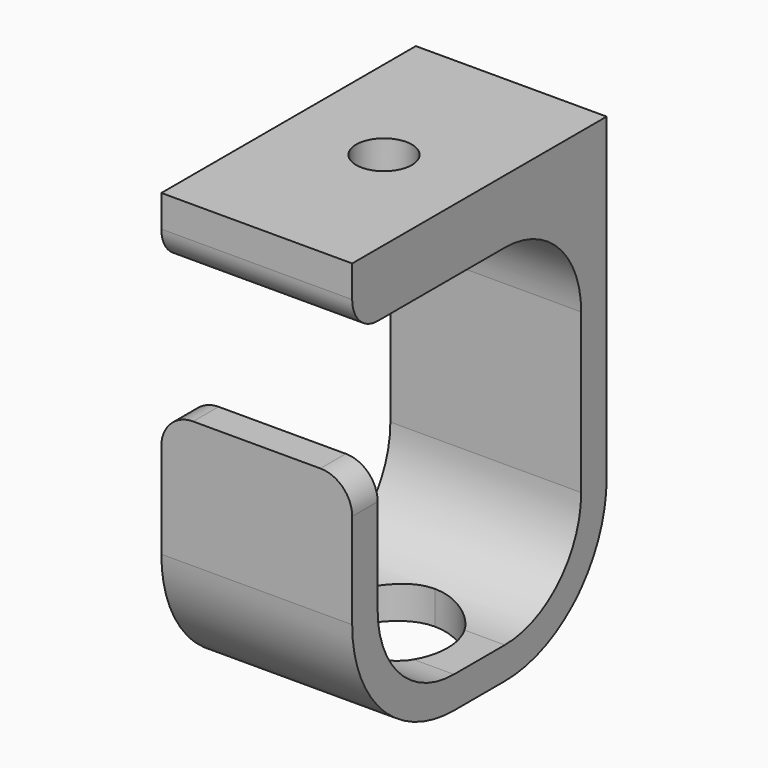
from build123d import *

# Parameters (mm, degrees)
F0_W     = 3.175
F0_H     = 6.35
F1_DEPTH = 9.525
F2_W     = 12.7
F2_H     = 6.35
F2_H_2   = 3.175
F3_DEPTH = 3.7207438789
F4_R     = 6.34999
F5_R     = 3.175
F6_R     = 2.778125
F7_DEPTH = 6.35
F8_R     = 2.778125
F9_DEPTH = 1.5875


# Not quite as in the source:
# - a fillet or chamfer is up to 0.001 mm smaller than in the source, because OpenCascade refuses the exact size
# - a feature names something its author has since deleted; it is built from what else it names


with BuildPart() as f1:
    # F0 (on Right) → F1 (new body, symmetric)
    with BuildSketch(Plane.YZ):
        with BuildLine():
            Line((31.75, 44.45), (3.175, 44.45))
            Line((3.175, 44.45), (3.175, 38.1))
            Line((3.175, 38.1), (19.05, 38.1))
            Line((19.05, 38.1), (28.575, 38.1))
            Line((28.575, 38.1), (28.575, 28.575))
            Line((28.575, 28.575), (28.575, 12.7))
            Line((28.575, 12.7), (28.575, 4.2997395874))
            ThreePointArc((28.575, 4.2997395874), (30.929762203, 8.2098719395), (31.75, 12.7))
            Line((31.75, 12.7), (31.75, 44.45))
        make_face()
        with Locations((1.5875, 41.275)):
            Rectangle(F0_W, F0_H)
        with BuildLine():
            Line((28.575, 38.1), (19.05, 38.1))
            ThreePointArc((19.05, 38.1), (25.7851920908, 35.3101920908), (28.575, 28.575))
            Line((28.575, 28.575), (28.575, 38.1))
        make_face()
        with BuildLine():
            ThreePointArc((27.4502604126, 3.175), (28.0302561211, 3.7197438789), (28.575, 4.2997395874))
            Line((28.575, 4.2997395874), (28.575, 12.7))
            ThreePointArc((28.575, 12.7), (25.7851920908, 5.9648079092), (19.05, 3.175))
            Line((19.05, 3.175), (27.4502604126, 3.175))
        make_face()
        with BuildLine():
            ThreePointArc((19.05, 0), (23.5401280605, 0.820237797), (27.4502604126, 3.175))
            Line((27.4502604126, 3.175), (19.05, 3.175))
            Line((19.05, 3.175), (12.7, 3.175))
            Line((12.7, 3.175), (4.2997395874, 3.175))
            ThreePointArc((4.2997395874, 3.175), (8.2098719395, 0.820237797), (12.7, 0))
            Line((12.7, 0), (19.05, 0))
        make_face()
        with BuildLine():
            ThreePointArc((12.7, 3.175), (5.9648079092, 5.9648079092), (3.175, 12.7))
            Line((3.175, 12.7), (3.175, 4.2997395874))
            ThreePointArc((3.175, 4.2997395874), (3.7197438789, 3.7197438789), (4.2997395874, 3.175))
            Line((4.2997395874, 3.175), (12.7, 3.175))
        make_face()
        with BuildLine():
            Line((3.175, 25.4), (0, 25.4))
            Line((0, 25.4), (0, 12.7))
            ThreePointArc((0, 12.7), (0.820237797, 8.2098719395), (3.175, 4.2997395874))
            Line((3.175, 4.2997395874), (3.175, 12.7))
            Line((3.175, 12.7), (3.175, 25.4))
        make_face()
    extrude(amount=F1_DEPTH, both=True)

    # F2 (on face) → F3 (cut, through all)
    with BuildSketch(Plane(origin=(0, 0, 0), x_dir=(1, 0, 0), z_dir=(0, 0, -1))):
        with Locations((0, -15.875)):
            Rectangle(F2_W, F2_H)
        with Locations((0, -11.1125)):
            Rectangle(F2_W, F2_H_2)
        with Locations((0, -20.6375)):
            Rectangle(F2_W, F2_H_2)
    extrude(amount=-F3_DEPTH, mode=Mode.SUBTRACT)

    # F4 (radius 6.35 in the source; OpenCascade refuses exactly that, so slightly less here)
    f4_edges = [f1.edges().sort_by_distance(p)[0] for p in [
        (-6.35, 22.225, 2.061511),
        (-6.35, 9.525, 2.061511),
        (6.35, 9.525, 2.061511),
        (6.35, 22.225, 2.061511),
    ]]
    fillet(f4_edges, radius=F4_R)

    # F5
    f5_edges = [f1.edges().sort_by_distance(p)[0] for p in [
        (0, 0, 38.1),
        (9.525, 1.5875, 25.4),
        (-9.525, 1.5875, 25.4),
    ]]
    fillet(f5_edges, radius=F5_R)

    # F6 (on face) → F7 (cut, through all)
    with BuildSketch(Plane.XY.offset(44.45)):
        with Locations((0, 15.875)):
            Circle(F6_R)
    extrude(amount=-F7_DEPTH, mode=Mode.SUBTRACT)

    # F8 (on face) → F9 (cut, symmetric)
    with BuildSketch(Plane(origin=(0, 0, 38.1), x_dir=(1, 0, 0), z_dir=(0, 0, -1))):
        with BuildLine():
            ThreePointArc((4.5597466007, -19.05), (5.3012737202, -17.5388542623), (5.55625, -15.875))
            ThreePointArc((5.55625, -15.875), (-1.6638542623, -10.5737262798), (-4.5597466007, -19.05))
            Line((-4.5597466007, -19.05), (4.5597466007, -19.05))
        make_face()
        with Locations((0, -15.875)):
            Circle(F8_R, mode=Mode.SUBTRACT)
        with BuildLine():
            Line((4.5597466007, -19.05), (-4.5597466007, -19.05))
            ThreePointArc((-4.5597466007, -19.05), (0, -21.43125), (4.5597466007, -19.05))
        make_face()
    extrude(amount=F9_DEPTH, both=True, mode=Mode.SUBTRACT)


solid = f1.part
